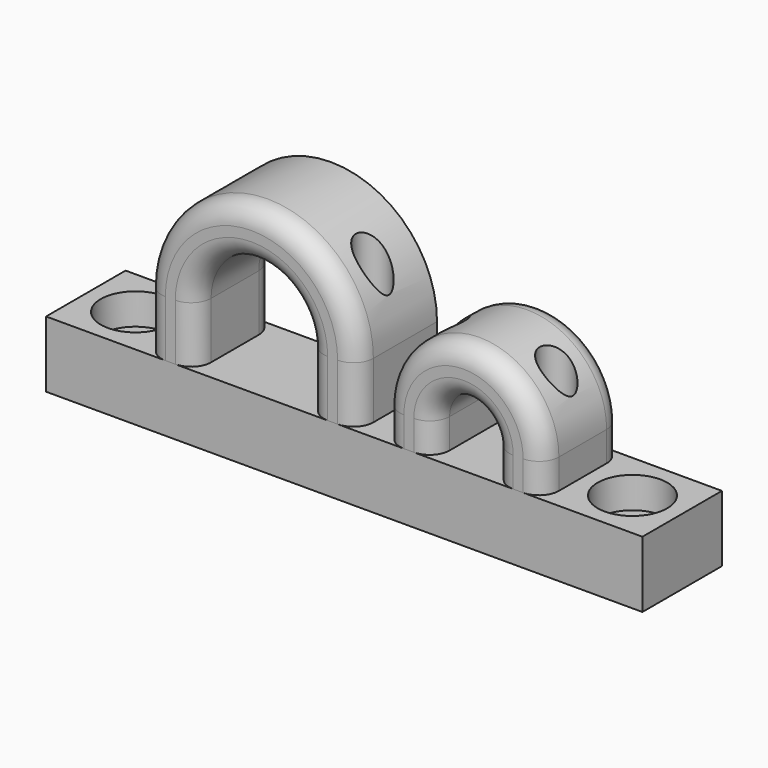
from build123d import *

# Parameters (mm, degrees)
F0_W     = 15
F0_H     = 10
F1_DEPTH = 7.5
F2_DEPTH = 7.5
F4_R     = 2.75
F5_DEPTH = 40
F6_DEPTH = 15
F7_DEPTH = 18
F4_R_2   = 5.25
F8_DEPTH = 29.2
F9_R     = 3
F9_2_R   = 3


with BuildPart() as f1:
    # F0 (on Front) → F1 (new body, symmetric)
    with BuildSketch(Plane.XZ):
        with Locations((-41.5, 5)):
            Rectangle(F0_W, F0_H)
        Polygon((-34, 0), (0, 0), (26, 0), (26, 10), (18.5, 10), (9.5, 10), (2.5, 10), (2, 10), (-2, 10), (-9.5, 10), (-26.5, 10), (-34, 10), align=None)
        with Locations((33.5, 5)):
            Rectangle(F0_W, F0_H)
    extrude(amount=F1_DEPTH, both=True)


with BuildPart() as f2:
    # F0 (on Front) → F2 (new body, symmetric)
    with BuildSketch(Plane.XZ):
        with BuildLine():
            Line((-34, 18.5), (-34, 10))
            Line((-34, 10), (-26.5, 10))
            Line((-26.5, 10), (-26.5, 18.5))
            ThreePointArc((-26.5, 18.5), (-18, 27), (-9.5, 18.5))
            Line((-9.5, 18.5), (-9.5, 10))
            Line((-9.5, 10), (-2, 10))
            Line((-2, 10), (-2, 18.5))
            ThreePointArc((-2, 18.5), (-18, 34.5), (-34, 18.5))
        make_face()
    extrude(amount=F2_DEPTH, both=True)


with BuildPart() as f2b:
    # F0 (on Front) → F2, piece 2 (new body, symmetric)
    with BuildSketch(Plane.XZ):
        with BuildLine():
            Line((18.5, 10), (26, 10))
            Line((26, 10), (26, 14.5))
            ThreePointArc((26, 14.5), (14, 26.5), (2, 14.5))
            Line((2, 14.5), (2, 10))
            Line((2, 10), (2.5, 10))
            Line((2.5, 10), (9.5, 10))
            Line((9.5, 10), (9.5, 14.5))
            ThreePointArc((9.5, 14.5), (14, 19), (18.5, 14.5))
            Line((18.5, 14.5), (18.5, 10))
        make_face()
    extrude(amount=F2_DEPTH, both=True)


with BuildPart() as f5_tool:
    # F4 (on offset) → F5 (new body)
    with BuildSketch(Plane.XY.offset(34.5)):
        with Locations((-41.5, 0)):
            Circle(F4_R)
        with BuildLine():
            ThreePointArc((36.25, 0), (33.5, 2.75), (30.75, 0))
            ThreePointArc((30.75, 0), (33.5, -2.75), (36.25, 0))
        make_face()
        with BuildLine():
            ThreePointArc((-7.25, 0), (-5.75, -1.5), (-4.25, 0))
            Line((-4.25, 0), (-5.75, 0))
            Line((-5.75, 0), (-7.25, 0))
        make_face()
        with BuildLine():
            Line((-5.75, 0), (-4.25, 0))
            ThreePointArc((-4.25, 0), (-5.75, 1.5), (-7.25, 0))
            Line((-7.25, 0), (-5.75, 0))
        make_face()
        with BuildLine():
            ThreePointArc((7.25, 0), (5.75, 1.5), (4.25, 0))
            Line((4.25, 0), (5.75, 0))
            Line((5.75, 0), (7.25, 0))
        make_face()
        with BuildLine():
            Line((5.75, 0), (4.25, 0))
            ThreePointArc((4.25, 0), (5.75, -1.5), (7.25, 0))
            Line((7.25, 0), (5.75, 0))
        make_face()
        with BuildLine():
            ThreePointArc((-31.75, 0), (-30.25, -1.5), (-28.75, 0))
            Line((-28.75, 0), (-30.25, 0))
            Line((-30.25, 0), (-31.75, 0))
        make_face()
        with BuildLine():
            Line((-30.25, 0), (-28.75, 0))
            ThreePointArc((-28.75, 0), (-30.25, 1.5), (-31.75, 0))
            Line((-31.75, 0), (-30.25, 0))
        make_face()
        with BuildLine():
            ThreePointArc((23.5, 0), (22, 1.5), (20.5, 0))
            Line((20.5, 0), (22, 0))
            Line((22, 0), (23.5, 0))
        make_face()
        with BuildLine():
            Line((22, 0), (20.5, 0))
            ThreePointArc((20.5, 0), (22, -1.5), (23.5, 0))
            Line((23.5, 0), (22, 0))
        make_face()
    extrude(amount=-F5_DEPTH)


with BuildPart() as f1_1:
    add(f1.part)

    # F5: cut by f5_tool
    add(f5_tool.part, mode=Mode.SUBTRACT)

    # F4 (on offset) → F8 (cut)
    with BuildSketch(Plane.XY.offset(34.5)):
        with Locations((-41.5, 0)):
            Circle(F4_R_2)
        with Locations((-41.5, 0)):
            Circle(F4_R, mode=Mode.SUBTRACT)
        with BuildLine():
            ThreePointArc((38.75, 0), (33.5, 5.25), (28.25, 0))
            ThreePointArc((28.25, 0), (33.5, -5.25), (38.75, 0))
        make_face()
        with BuildLine():
            ThreePointArc((36.25, 0), (33.5, -2.75), (30.75, 0))
            ThreePointArc((30.75, 0), (33.5, 2.75), (36.25, 0))
        make_face(mode=Mode.SUBTRACT)
    extrude(amount=-F8_DEPTH, mode=Mode.SUBTRACT)


with BuildPart() as f2_1:
    add(f2.part)

    # F5: cut by f5_tool
    add(f5_tool.part, mode=Mode.SUBTRACT)


with BuildPart() as f2b_1:
    add(f2b.part)

    # F5: cut by f5_tool
    add(f5_tool.part, mode=Mode.SUBTRACT)


with BuildPart() as f6_tool:
    # F4 (on offset) → F6 (new body)
    with BuildSketch(Plane.XY.offset(34.5)):
        with BuildLine():
            ThreePointArc((-32.75, 0), (-30.25, -2.5), (-27.75, 0))
            Line((-27.75, 0), (-28.75, 0))
            ThreePointArc((-28.75, 0), (-30.25, -1.5), (-31.75, 0))
            Line((-31.75, 0), (-32.75, 0))
        make_face()
        with BuildLine():
            Line((-28.75, 0), (-27.75, 0))
            ThreePointArc((-27.75, 0), (-30.25, 2.5), (-32.75, 0))
            Line((-32.75, 0), (-31.75, 0))
            ThreePointArc((-31.75, 0), (-30.25, 1.5), (-28.75, 0))
        make_face()
        with BuildLine():
            ThreePointArc((-8.25, 0), (-5.75, -2.5), (-3.25, 0))
            Line((-3.25, 0), (-4.25, 0))
            ThreePointArc((-4.25, 0), (-5.75, -1.5), (-7.25, 0))
            Line((-7.25, 0), (-8.25, 0))
        make_face()
        with BuildLine():
            Line((-4.25, 0), (-3.25, 0))
            ThreePointArc((-3.25, 0), (-5.75, 2.5), (-8.25, 0))
            Line((-8.25, 0), (-7.25, 0))
            ThreePointArc((-7.25, 0), (-5.75, 1.5), (-4.25, 0))
        make_face()
        with BuildLine():
            ThreePointArc((24.5, 0), (22, 2.5), (19.5, 0))
            Line((19.5, 0), (20.5, 0))
            ThreePointArc((20.5, 0), (22, 1.5), (23.5, 0))
            Line((23.5, 0), (24.5, 0))
        make_face()
        with BuildLine():
            ThreePointArc((8.25, 0), (5.75, 2.5), (3.25, 0))
            Line((3.25, 0), (4.25, 0))
            ThreePointArc((4.25, 0), (5.75, 1.5), (7.25, 0))
            Line((7.25, 0), (8.25, 0))
        make_face()
    extrude(amount=-F6_DEPTH)


with BuildPart() as f2_2:
    add(f2_1.part)

    # F6: cut by f6_tool
    add(f6_tool.part, mode=Mode.SUBTRACT)

    # F9
    f9_edges = [f2_2.edges().sort_by_distance(p)[0] for p in [
        (-18, -7.5, 34.5),
        (-18, -7.5, 27),
        (-18, 7.5, 27),
        (-34, -7.5, 14.25),
        (-9.5, 7.5, 14.25),
        (-9.5, -7.5, 14.25),
        (-26.5, 7.5, 14.25),
        (-26.5, -7.5, 14.25),
        (-2, -7.5, 14.25),
    ]]
    fillet(f9_edges, radius=F9_R)


with BuildPart() as f2b_2:
    add(f2b_1.part)

    # F6: cut by f6_tool
    add(f6_tool.part, mode=Mode.SUBTRACT)

    # F4 (on offset) → F7 (cut)
    with BuildSketch(Plane.XY.offset(34.5)):
        with BuildLine():
            ThreePointArc((24.5, 0), (22, 2.5), (19.5, 0))
            Line((19.5, 0), (20.5, 0))
            ThreePointArc((20.5, 0), (22, 1.5), (23.5, 0))
            Line((23.5, 0), (24.5, 0))
        make_face()
        with BuildLine():
            Line((20.5, 0), (19.5, 0))
            ThreePointArc((19.5, 0), (22, -2.5), (24.5, 0))
            Line((24.5, 0), (23.5, 0))
            ThreePointArc((23.5, 0), (22, -1.5), (20.5, 0))
        make_face()
        with BuildLine():
            ThreePointArc((8.25, 0), (5.75, 2.5), (3.25, 0))
            Line((3.25, 0), (4.25, 0))
            ThreePointArc((4.25, 0), (5.75, 1.5), (7.25, 0))
            Line((7.25, 0), (8.25, 0))
        make_face()
        with BuildLine():
            Line((4.25, 0), (3.25, 0))
            ThreePointArc((3.25, 0), (5.75, -2.5), (8.25, 0))
            Line((8.25, 0), (7.25, 0))
            ThreePointArc((7.25, 0), (5.75, -1.5), (4.25, 0))
        make_face()
    extrude(amount=-F7_DEPTH, mode=Mode.SUBTRACT)

    # F9#2
    f9_2_edges = [f2b_2.edges().sort_by_distance(p)[0] for p in [
        (14, -7.5, 26.5),
        (14, -7.5, 19),
        (14, 7.5, 19),
        (14, 7.5, 26.5),
        (18.5, 7.5, 12.25),
        (18.5, -7.5, 12.25),
        (26, 7.5, 12.25),
        (26, -7.5, 12.25),
        (2, 7.5, 12.25),
        (2, -7.5, 12.25),
        (9.5, -7.5, 12.25),
        (9.5, 7.5, 12.25),
    ]]
    fillet(f9_2_edges, radius=F9_2_R)


solid = Compound([f1_1.part, f2_2.part, f2b_2.part])
